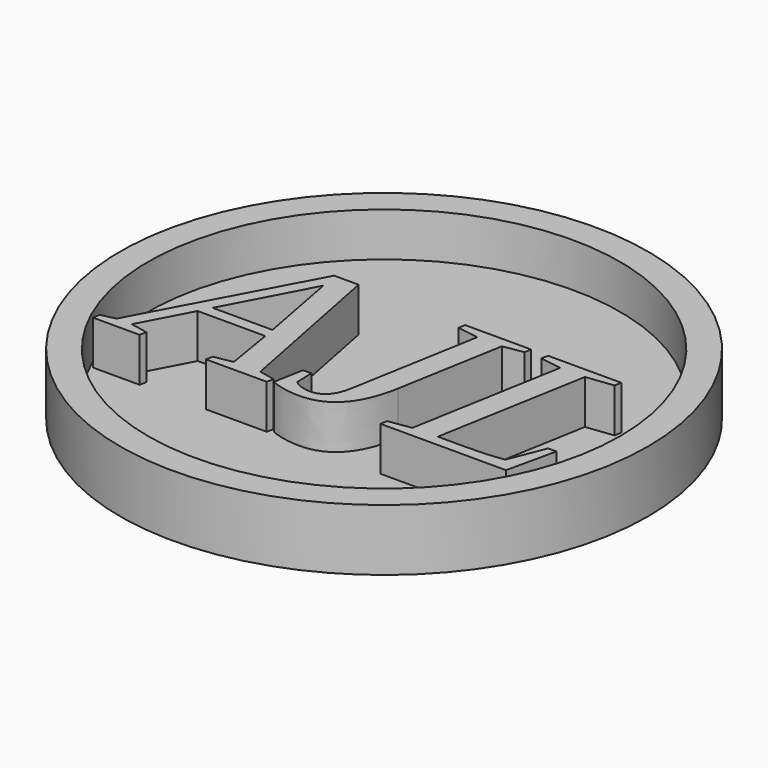
from build123d import *

# Parameters (mm, degrees)
F0_R         = 15
F1_DEPTH     = 1
F2_TEXT_SIZE = 14.8960940043
F3_DEPTH     = 2.5
F4_R         = 15
F4_R_2       = 13.4137742962
F5_DEPTH     = 2.5


# Not quite as in the source:
# - Text() gives the source's letters only with a copy of the font that has no kerning and outlines rounded to 1/6400 em; it was checked with that copy


with BuildPart() as f1:
    # F0 (on Top) → F1 (new body)
    with BuildSketch(Plane.XY):
        Circle(F0_R)
    extrude(amount=F1_DEPTH)

    # F2 (on face) → F3 (join)
    with BuildSketch(Plane.XY.offset(1)):
        with Locations((-11.1662395066, -5.7152841187)):
            Text('AJL', F2_TEXT_SIZE, font='Tinos', font_style=FontStyle.ITALIC, text_align=(TextAlign.LEFT, TextAlign.BOTTOM))
    extrude(amount=F3_DEPTH)

    # F4 (on face) → F5 (join)
    with BuildSketch(Plane.XY.offset(1)):
        Circle(F4_R)
        Circle(F4_R_2, mode=Mode.SUBTRACT)
    extrude(amount=F5_DEPTH)


solid = f1.part
